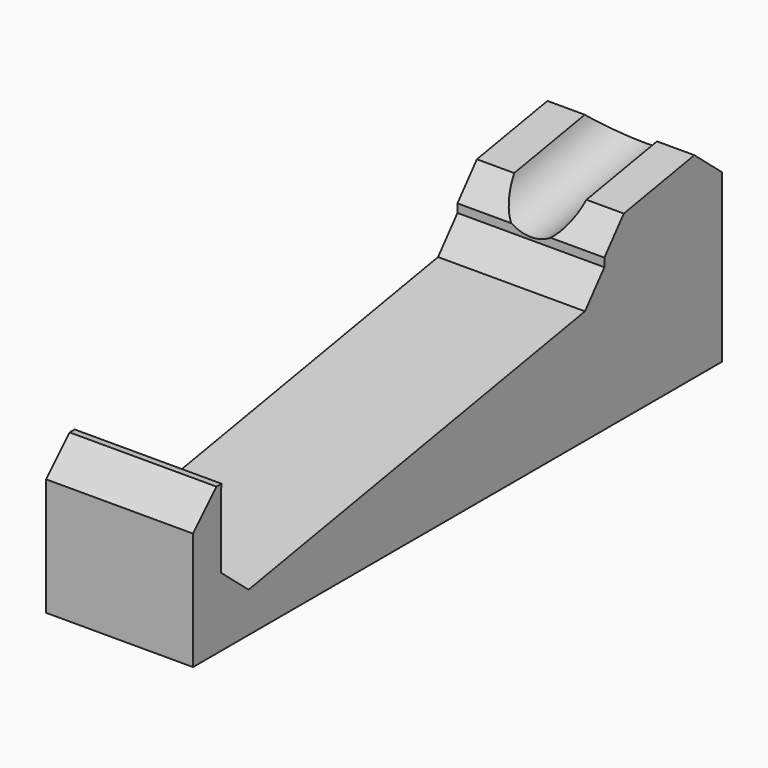
from build123d import *

# Parameters (mm, degrees)
F1_DEPTH     = 12.7
F3_R         = 6.35
F4_DEPTH     = 104.14
F5_T1_DEPTH  = 25.4
F5_T3_DEPTH  = 51.5282991577
F5_T5_DEPTH  = 37.3912990947
F5_T7_DEPTH  = 28.55897566
F5_T9_DEPTH  = 28.55897566
F5_T11_DEPTH = 37.3912990947


# Not quite as in the source:
# - a fillet or chamfer that OpenCascade refuses, or shapes differently, is made with other operations: its cross-section is extruded or revolved along the edge and cut away or added


with BuildPart() as f1:
    # F0 (on Right) → F1 (new body, symmetric)
    with BuildSketch(Plane.YZ):
        Polygon((-114.3, 25.4), (-114.3, 0), (0, 0), (0, 34.925), (-25.4, 30.44629469), (-25.4, 20.4565655141), (-108.2500742316, 5.8478620733), (-108.2500742316, 24.8292279061), (-108.1259697676, 24.8511108716), (-108.1259697676, 25.4), align=None)
    extrude(amount=F1_DEPTH, both=True)

    # F3 (on face) → F4 (cut)
    with BuildSketch(Plane(origin=(0, 5.9725267528, 1.0531176095), x_dir=(1, 0, 0), z_dir=(0, -0.984807753, -0.1736481777))):
        with Locations((0, 35.56)):
            Circle(F3_R)
    extrude(amount=F4_DEPTH, mode=Mode.SUBTRACT)

    # F5: chamfer of 5.08 on 7 edges, made by hand

    # F5_s2 → F5_t1 (join)
    with BuildSketch(Plane.YZ.offset(-12.7)):
        Polygon((-25.4, 24.7191916404), (-29.5978672575, 19.7163682551), (-25.4, 20.4565655141), align=None)
        Polygon((-102.2879414891, 6.8991469384), (-108.2500742316, 11.9019703237), (-108.2500742316, 5.8478620733), align=None)
    extrude(amount=F5_T1_DEPTH)

    # F5_s4 → F5_t3 (cut)
    with BuildSketch(Plane.YZ.offset(-25.7641495789)):
        Polygon((-114.3, 20.32), (-109.22, 25.4), (-114.3, 25.4), align=None)
    extrude(amount=F5_T3_DEPTH, mode=Mode.SUBTRACT)

    # F5_s6 → F5_t5 (cut)
    with BuildSketch(Plane.YZ.offset(-28.1667031257)):
        Polygon((0, 28.8708917496), (-5.9621327425, 33.8737151349), (0, 34.925), align=None)
    extrude(amount=F5_T5_DEPTH, mode=Mode.SUBTRACT)

    # F5_s8 → F5_t7 (cut)
    with BuildSketch(Plane.YZ.offset(-4.8084342517)):
        Polygon((-25.4, 26.1836685636), (-21.2021327425, 31.1864919489), (-25.4, 30.44629469), align=None)
    extrude(amount=F5_T7_DEPTH, mode=Mode.SUBTRACT)

    # F5_s10 → F5_t9 (cut)
    with BuildSketch(Plane.YZ.offset(-23.7505414084)):
        Polygon((-21.2021327425, 31.1864919489), (-25.4, 26.1836685636), (-25.4, 30.44629469), align=None)
    extrude(amount=F5_T9_DEPTH, mode=Mode.SUBTRACT)

    # F5_s12 → F5_t11 (cut)
    with BuildSketch(Plane.YZ.offset(-9.224595969)):
        Polygon((0, 28.8708917496), (-5.9621327425, 33.8737151349), (0, 34.925), align=None)
    extrude(amount=F5_T11_DEPTH, mode=Mode.SUBTRACT)


solid = f1.part
